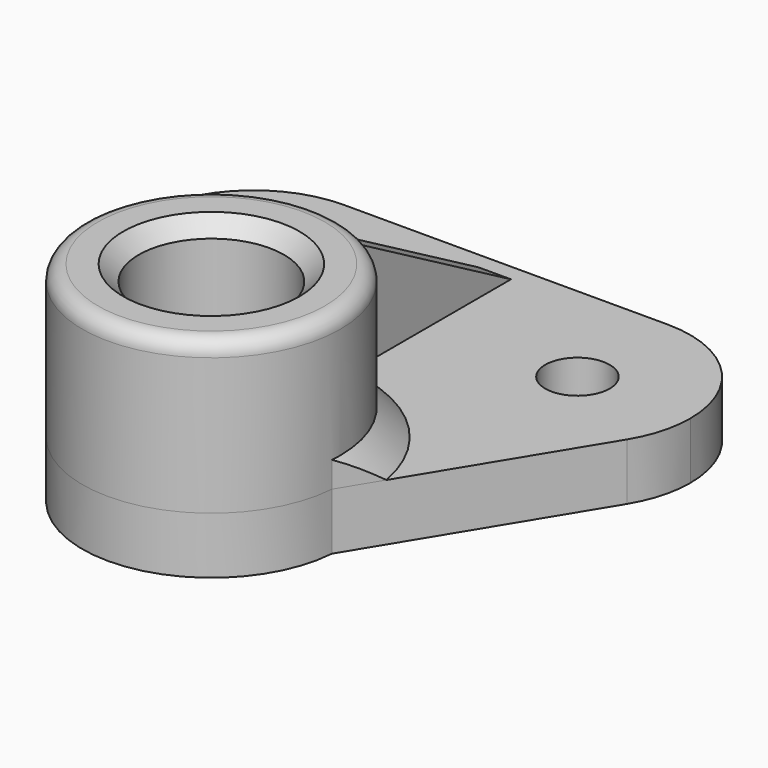
from build123d import *

# Parameters (mm, degrees)
F0_R         = 14.3129
F0_R_2       = 6.35
F1_DEPTH     = 11.176
F2_R         = 25.4
F2_R_2       = 14.2875
F3_DEPTH     = 41.148
F4_R         = 3.048
F6_DEPTH     = 26.67
F8_DEPTH     = 36.576
F9_SIZE      = 3.048
F10_T4_ANGLE = 146.2844316289
F10_T9_ANGLE = 141.7779247294


# Not quite as in the source:
# - a fillet or chamfer that OpenCascade refuses, or shapes differently, is made with other operations: its cross-section is extruded or revolved along the edge and cut away or added


with BuildPart() as f1:
    # F0 (on Top) → F1 (new body)
    with BuildSketch(Plane.XY):
        with BuildLine():
            ThreePointArc((25.3215518154, -1.9947465156), (25.3803803765, -0.9981442505), (25.4, 0))
            ThreePointArc((25.4, 0), (-0.9981442505, 25.3803803765), (-25.3215518154, -1.9947465156))
            ThreePointArc((-25.3215518154, -1.9947465156), (0, -25.4), (25.3215518154, -1.9947465156))
        make_face()
        Circle(F0_R, mode=Mode.SUBTRACT)
        with BuildLine():
            ThreePointArc((-25.3215518154, -1.9947465156), (-0.9981442505, 25.3803803765), (25.4, 0))
            ThreePointArc((25.4, 0), (25.3803803765, -0.9981442505), (25.3215518154, -1.9947465156))
            Line((25.3215518154, -1.9947465156), (50.3921391886, 39.2574286123))
            ThreePointArc((50.3921391886, 39.2574286123), (12.0283500327, 39.9046575109), (31.3995177065, 73.025))
            Line((31.3995177065, 73.025), (-32.3313889886, 73.025))
            ThreePointArc((-32.3313889886, 73.025), (-16.6159407767, 66.5154482119), (-10.1063889886, 50.8))
            ThreePointArc((-10.1063889886, 50.8), (-26.1628636627, 29.4481869551), (-51.1322535829, 38.9476535864))
            Line((-51.1322535829, 38.9476535864), (-25.3215518154, -1.9947465156))
        make_face()
        with BuildLine():
            ThreePointArc((-32.3313889886, 73.025), (-51.7912068711, 61.5362057068), (-51.1322535829, 38.9476535864))
            ThreePointArc((-51.1322535829, 38.9476535864), (-26.1628636627, 29.4481869551), (-10.1063889886, 50.8))
            ThreePointArc((-10.1063889886, 50.8), (-16.6159407767, 66.5154482119), (-32.3313889886, 73.025))
        make_face()
        with Locations((-32.3313889886, 50.8)):
            Circle(F0_R_2, mode=Mode.SUBTRACT)
        with BuildLine():
            ThreePointArc((31.3995177065, 73.025), (12.0283500327, 39.9046575109), (50.3921391886, 39.2574286123))
            ThreePointArc((50.3921391886, 39.2574286123), (52.8011722855, 44.8066865357), (53.6245177065, 50.8))
            ThreePointArc((53.6245177065, 50.8), (47.1149659184, 66.5154482119), (31.3995177065, 73.025))
        make_face()
        with Locations((31.3995177065, 50.8)):
            Circle(F0_R_2, mode=Mode.SUBTRACT)
    extrude(amount=F1_DEPTH)

    # F2 (on Top) → F3 (join)
    with BuildSketch(Plane.XY):
        Circle(F2_R)
        Circle(F2_R_2, mode=Mode.SUBTRACT)
    extrude(amount=F3_DEPTH)

    # F4
    f4_edges = [f1.edges().sort_by_distance(p)[0] for p in [
        (-25.4, 0, 41.148),
    ]]
    fillet(f4_edges, radius=F4_R)

    # F5 (on face) → F6 (join)
    with BuildSketch(Plane.XY.offset(11.176)):
        with BuildLine():
            Line((3.175, 69.723), (0, 69.723))
            Line((0, 69.723), (-3.175, 69.723))
            Line((-3.175, 69.723), (-3.175, 25.2007812379))
            ThreePointArc((-3.175, 25.2007812379), (0, 25.4), (3.175, 25.2007812379))
            Line((3.175, 25.2007812379), (3.175, 69.723))
        make_face()
    extrude(amount=F6_DEPTH)

    # F7 (on face) → F8 (cut)
    with BuildSketch(Plane.YZ.offset(3.175)):
        Polygon((25.2007812379, 37.846), (25.3999978304, 36.3681837916), (69.723, 11.176), (69.723, 37.846), align=None)
    extrude(amount=-F8_DEPTH, mode=Mode.SUBTRACT)

    # F9
    f9_edges = [f1.edges().sort_by_distance(p)[0] for p in [
        (-14.2875, 0, 41.148),
    ]]
    chamfer(f9_edges, length=F9_SIZE)

    # F10: chamfer of 5.08 on 3 edges, made by hand


with BuildPart() as f10_tool2:
    # F10_s3 → F10_t4 (revolve)
    with BuildSketch(Plane(origin=(0, 0, 0), x_dir=(0, 0, 1), z_dir=(0.55897189, -0.8291866052, 0))):
        Polygon((16.256, 25.4), (11.176, 30.48), (11.176, 25.4), align=None)
    revolve(axis=Axis((0, 0, 11.176), (0, 0, -1)), revolution_arc=F10_T4_ANGLE)

    split(bisect_by=Plane(origin=(-19.0200600063, -11.9905304818, 0), x_dir=(0, 0, 1), z_dir=(0.8459331651, 0.5332889275, 0)), keep=Keep.TOP)


with BuildPart() as f1_1:
    add(f1.part)

    # F10_t1: union F10_tool2
    add(f10_tool2.part)


with BuildPart() as f10_tool7:
    # F10_s8 → F10_t9 (revolve)
    with BuildSketch(Plane(origin=(0, 0, 0), x_dir=(0, 0, 1), z_dir=(-0.9252190928, -0.3794333016, 0))):
        Polygon((16.256, 25.4), (11.176, 30.48), (11.176, 25.4), align=None)
    revolve(axis=Axis((0, 0, 11.176), (0, 0, -1)), revolution_arc=F10_T9_ANGLE)

    split(bisect_by=Plane(origin=(19.3769924359, -11.7761689023, 0), x_dir=(0, 0, 1), z_dir=(-0.8545611465, 0.5193507936, 0)), keep=Keep.TOP)


with BuildPart() as f1_2:
    add(f1_1.part)

    # F10_t6: union F10_tool7
    add(f10_tool7.part)


solid = f1_2.part
